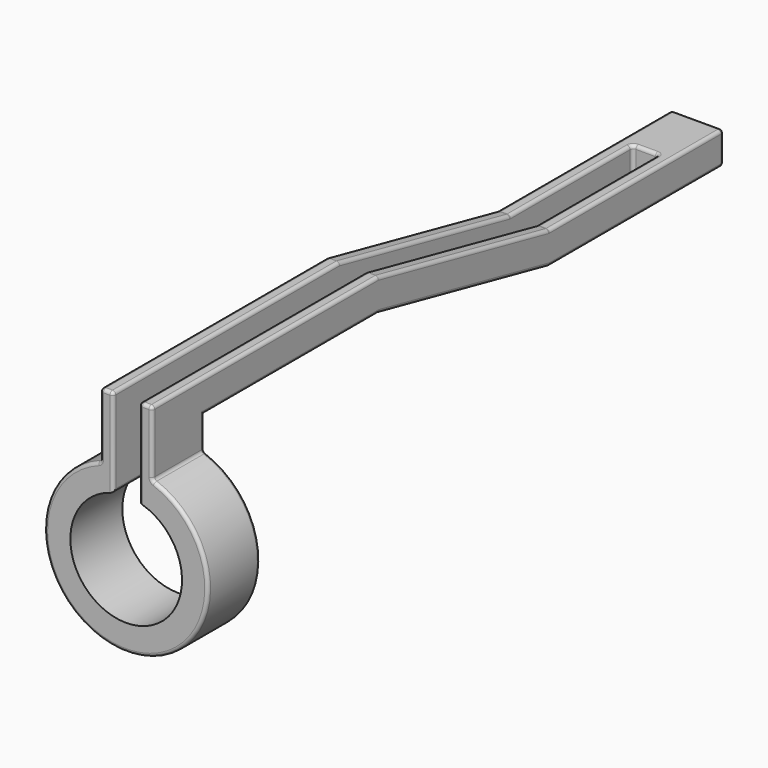
from build123d import *

# Parameters (mm, degrees)
F0_R          = 6.3
F1_DEPTH      = 5
F2_R          = 4.3
F3_DEPTH      = 5
F4_W          = 4
F4_H          = 5
F5_DEPTH      = 5
F7_DEPTH      = 4
F9_DEPTH      = 50
F10_F1_R      = 0.25
F10_F2_R      = 0.25
F11_T1_DEPTH  = 0.5
F11_T3_DEPTH  = 0.5
F11_S7_W      = 0.25
F11_S7_H      = 0.25
F11_T8_DEPTH  = 0.25
F11_S13_W     = 0.25
F11_S13_H     = 0.25
F11_T14_DEPTH = 0.25
F11_S19_W     = 0.25
F11_S19_H     = 0.25
F11_T20_DEPTH = 0.25
F11_S25_W     = 0.25
F11_S25_H     = 0.25
F11_T26_DEPTH = 0.25


# Not quite as in the source:
# - a fillet or chamfer that OpenCascade refuses, or shapes differently, is made with other operations: its cross-section is extruded or revolved along the edge and cut away or added


with BuildPart() as f1:
    # F0 (on Front) → F1 (new body)
    with BuildSketch(Plane.XZ):
        Circle(F0_R)
    extrude(amount=F1_DEPTH)

    # F2 (on face) → F3 (cut, through all)
    with BuildSketch(Plane.XZ.offset(5)):
        Circle(F2_R)
    extrude(amount=-F3_DEPTH, mode=Mode.SUBTRACT)

    # F4 (on face) → F5 (join)
    with BuildSketch(Plane.XZ.offset(5)):
        with Locations((0, 8.4741108125)):
            Rectangle(F4_W, F4_H)
    extrude(amount=-F5_DEPTH)

    # F6 (on face) → F7 (join, through all)
    with BuildSketch(Plane.YZ.offset(2)):
        Polygon((16.7896201938, 10.9741108125), (0, 10.9741108125), (0, 8.4741108125), (16.7896201938, 8.4741108125), (33.2103798062, 4.9741108125), (50, 4.9741108125), (50, 7.4741108125), (33.2103798062, 7.4741108125), align=None)
    extrude(amount=-F7_DEPTH)

    # F8 (on face) → F9 (cut)
    with BuildSketch(Plane.XZ.offset(5)):
        with BuildLine():
            Line((1, 4.1821047333), (1, 10.9741108125))
            Line((1, 10.9741108125), (-1, 10.9741108125))
            Line((-1, 10.9741108125), (-1, 4.1821047333))
            ThreePointArc((-1, 4.1821047333), (0, 4.3), (1, 4.1821047333))
        make_face()
    extrude(amount=-F9_DEPTH, mode=Mode.SUBTRACT)

    # F10: fillet of radius 0.25 on 50 edges, made by hand

    # F10_f1
    f10_f1_edges = [f1.edges().sort_by_distance(p)[0] for p in [
        (-1.5, 0, 8.4741108125),
        (-1.5, 16.7896201938, 8.4741108125),
        (-2, -2.5, 5.9741108125),
        (-1, 45, 6.2241108125),
        (1, 45, 6.2241108125),
        (2, -2.5, 5.9741108125),
        (1.5, 33.2103798062, 7.4741108125),
        (-1.5, 33.2103798062, 7.4741108125),
    ]]
    fillet(f10_f1_edges, radius=F10_F1_R)

    # F10_f2
    f10_f2_edges = [f1.edges().sort_by_distance(p)[0] for p in [
        (-2, 8.5066365047, 8.4741108125),
        (-2, 0, 7.1877667061),
        (-1, 0, 6.2031077729),
        (-1, 8.5066365047, 8.4741108125),
        (-2, 5.8948100969, 10.9741108125),
        (-2, 24.9871158258, 9.2268570076),
        (-2, 41.6183634953, 7.4741108125),
        (-2, 50, 6.2241108125),
        (-2, 41.6051899031, 4.9741108125),
        (-2, 25.0128841742, 6.7213646174),
        (-2, -5, 8.5627667061),
        (-1, 25.0128841742, 6.7213646174),
        (-1.5, 33.2103798062, 4.9741108125),
        (-1, -5, 7.5781077729),
        (-1, -2.5, 4.1821047333),
        (-1, 38.9801899031, 4.9741108125),
        (-1, 38.9933634953, 7.4741108125),
        (-1, 24.9871158258, 9.2268570076),
        (-1, 5.8948100969, 10.9741108125),
        (1, -5, 7.5781077729),
        (1, 5.8948100969, 10.9741108125),
        (1, 24.9871158258, 9.2268570076),
        (1, 38.9933634953, 7.4741108125),
        (1, 38.9801899031, 4.9741108125),
        (1, 25, 6.7241108125),
        (1, 8.3948100969, 8.4741108125),
        (1, 0, 6.3281077729),
        (1, -2.5, 4.1821047333),
        (2, 41.6051899031, 4.9741108125),
        (0, 50, 4.9741108125),
        (0, 45, 4.9741108125),
        (1.5, 33.2103798062, 4.9741108125),
        (2, 0, 7.3127667061),
        (2, 8.3948100969, 8.4741108125),
        (2, 25, 6.7241108125),
        (2, 50, 6.2241108125),
        (2, 41.6183634953, 7.4741108125),
        (2, 24.9871158258, 9.2268570076),
        (2, 5.8948100969, 10.9741108125),
        (2, -5, 8.5627667061),
        (0, 45, 7.4741108125),
        (0, 50, 7.4741108125),
        (-0.9267766953, 44.9267766953, 7.4741108125),
        (0.9267766953, 44.9267766953, 7.4741108125),
        (2.0450982362, -5, 6.0081910837),
        (2, 33.2105249149, 7.4754877017),
        (2.0450982362, 0, 6.0081910837),
        (0.9267766953, 44.9267766953, 4.9741108125),
        (-0.9267766953, 44.9267766953, 4.9741108125),
        (1, 33.2105249149, 7.4754877017),
        (-1, 33.2105249149, 7.4754877017),
        (-1, 16.7894750851, 8.4727339233),
        (-2.0450982362, -5, 6.0081910837),
        (-2, 16.7894750851, 8.4727339233),
        (-2, 33.2105249149, 7.4754877017),
        (-1, 0.0732233047, 8.4008875078),
        (-2, 0.0732233047, 8.4008875078),
        (-2.0450982362, 0, 6.0081910837),
    ]]
    fillet(f10_f2_edges, radius=F10_F2_R)

    # F11: fillet of radius 0.25 on 2 edges, made by hand

    # F11_s2 → F11_t1 (cut)
    with BuildSketch(Plane.YZ.offset(1.25)):
        with BuildLine():
            ThreePointArc((-5, 10.7241108125), (-4.9267766953, 10.9008875078), (-4.75, 10.9741108125))
            Line((-4.75, 10.9741108125), (-5, 10.9741108125))
            Line((-5, 10.9741108125), (-5, 10.7241108125))
        make_face()
    extrude(amount=F11_T1_DEPTH, mode=Mode.SUBTRACT)

    # F11_s4 → F11_t3 (cut)
    with BuildSketch(Plane.YZ.offset(-1.75)):
        with BuildLine():
            ThreePointArc((-5, 10.7241108125), (-4.9267766953, 10.9008875078), (-4.75, 10.9741108125))
            Line((-4.75, 10.9741108125), (-5, 10.9741108125))
            Line((-5, 10.9741108125), (-5, 10.7241108125))
        make_face()
    extrude(amount=F11_T3_DEPTH, mode=Mode.SUBTRACT)


with BuildPart() as f11_tool6:
    # F11_s7 → F11_t8 (new body)
    with BuildSketch(Plane.XZ.offset(4.75)):
        with Locations((-1.125, 10.8491108125)):
            Rectangle(F11_S7_W, F11_S7_H)
    extrude(amount=F11_T8_DEPTH)

    # F11_s9 → F11_t10 (revolve, cut)
    with BuildSketch(Plane(origin=(-1.25, -4.75, 10.7241108125), x_dir=(-0.7071067812, 0, -0.7071067812), z_dir=(-0.7071067812, 0, 0.7071067812))):
        with BuildLine():
            ThreePointArc((0, -0.25), (0.25, 0), (0, 0.25))
            Line((0, 0.25), (0, -0.25))
        make_face()
    revolve(axis=Axis((-1.25, -4.75, 10.7241108125), (0, -1, 0)), mode=Mode.SUBTRACT)


with BuildPart() as f1_1:
    add(f1.part)

    # F11_t5: cut F11_tool6
    add(f11_tool6.part, mode=Mode.SUBTRACT)


with BuildPart() as f11_tool12:
    # F11_s13 → F11_t14 (new body)
    with BuildSketch(Plane.XZ.offset(4.75)):
        with Locations((-1.875, 10.8491108125)):
            Rectangle(F11_S13_W, F11_S13_H)
    extrude(amount=F11_T14_DEPTH)

    # F11_s15 → F11_t16 (revolve, cut)
    with BuildSketch(Plane(origin=(-1.75, -4.75, 10.7241108125), x_dir=(0.7071067812, 0, -0.7071067812), z_dir=(-0.7071067812, 0, -0.7071067812))):
        with BuildLine():
            ThreePointArc((0, -0.25), (0.25, 0), (0, 0.25))
            Line((0, 0.25), (0, -0.25))
        make_face()
    revolve(axis=Axis((-1.75, -4.75, 10.7241108125), (0, -1, 0)), mode=Mode.SUBTRACT)


with BuildPart() as f1_2:
    add(f1_1.part)

    # F11_t11: cut F11_tool12
    add(f11_tool12.part, mode=Mode.SUBTRACT)


with BuildPart() as f11_tool18:
    # F11_s19 → F11_t20 (new body)
    with BuildSketch(Plane.XZ.offset(4.75)):
        with Locations((1.875, 10.8491108125)):
            Rectangle(F11_S19_W, F11_S19_H)
    extrude(amount=F11_T20_DEPTH)

    # F11_s21 → F11_t22 (revolve, cut)
    with BuildSketch(Plane(origin=(1.75, -4.75, 10.7241108125), x_dir=(-0.7071067812, 0, -0.7071067812), z_dir=(-0.7071067812, 0, 0.7071067812))):
        with BuildLine():
            ThreePointArc((0, -0.25), (0.25, 0), (0, 0.25))
            Line((0, 0.25), (0, -0.25))
        make_face()
    revolve(axis=Axis((1.75, -4.75, 10.7241108125), (0, -1, 0)), mode=Mode.SUBTRACT)


with BuildPart() as f1_3:
    add(f1_2.part)

    # F11_t17: cut F11_tool18
    add(f11_tool18.part, mode=Mode.SUBTRACT)


with BuildPart() as f11_tool24:
    # F11_s25 → F11_t26 (new body)
    with BuildSketch(Plane.XZ.offset(4.75)):
        with Locations((1.125, 10.8491108125)):
            Rectangle(F11_S25_W, F11_S25_H)
    extrude(amount=F11_T26_DEPTH)

    # F11_s27 → F11_t28 (revolve, cut)
    with BuildSketch(Plane(origin=(1.25, -4.75, 10.7241108125), x_dir=(0.7071067812, 0, -0.7071067812), z_dir=(-0.7071067812, 0, -0.7071067812))):
        with BuildLine():
            ThreePointArc((0, -0.25), (0.25, 0), (0, 0.25))
            Line((0, 0.25), (0, -0.25))
        make_face()
    revolve(axis=Axis((1.25, -4.75, 10.7241108125), (0, -1, 0)), mode=Mode.SUBTRACT)


with BuildPart() as f1_4:
    add(f1_3.part)

    # F11_t23: cut F11_tool24
    add(f11_tool24.part, mode=Mode.SUBTRACT)


solid = f1_4.part
